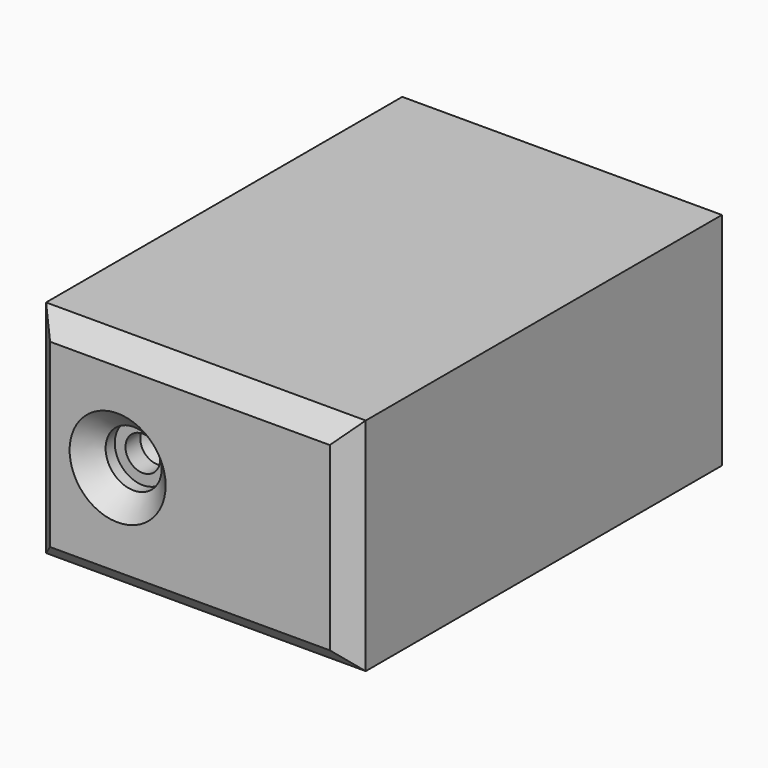
from build123d import *

# Parameters (mm, degrees)
F0_W           = 81.2892764807
F0_H           = 56.1117217876
F1_DEPTH       = 118.29543
F3_D           = 8.8
F3_DEPTH       = 12.7
F3_CBORE_D     = 14.25
F3_CBORE_DEPTH = 8
F3_TIP         = 2.6437867237
F4_SIZE        = 5.08


with BuildPart() as f1:
    # F0 (on Front) → F1 (new body)
    with BuildSketch(Plane.XZ):
        with Locations((12.407310307, -23.1582082342)):
            Rectangle(F0_W, F0_H)
    extrude(amount=F1_DEPTH)

    # F3
    with Locations(Plane.XZ.offset(118.29543)):
        with Locations((-5.9798196889, -22.842913866)):
            CounterBoreHole(F3_D / 2, F3_CBORE_D / 2, F3_CBORE_DEPTH, depth=F3_DEPTH)
            with Locations((0, 0, -(F3_DEPTH + F3_TIP / 2))):  # 118° drill point
                Cone(0, F3_D / 2, F3_TIP, mode=Mode.SUBTRACT)

    # F4
    f4_edges = [f1.edges().sort_by_distance(p)[0] for p in [
        (12.40731, -118.29543, 4.897653),
        (53.051949, -118.29543, -23.158208),
        (-28.237328, -118.29543, -23.158208),
        (12.40731, -118.29543, -51.214069),
        (-13.10482, -118.29543, -22.842914),
    ]]
    chamfer(f4_edges, length=F4_SIZE)


solid = f1.part
